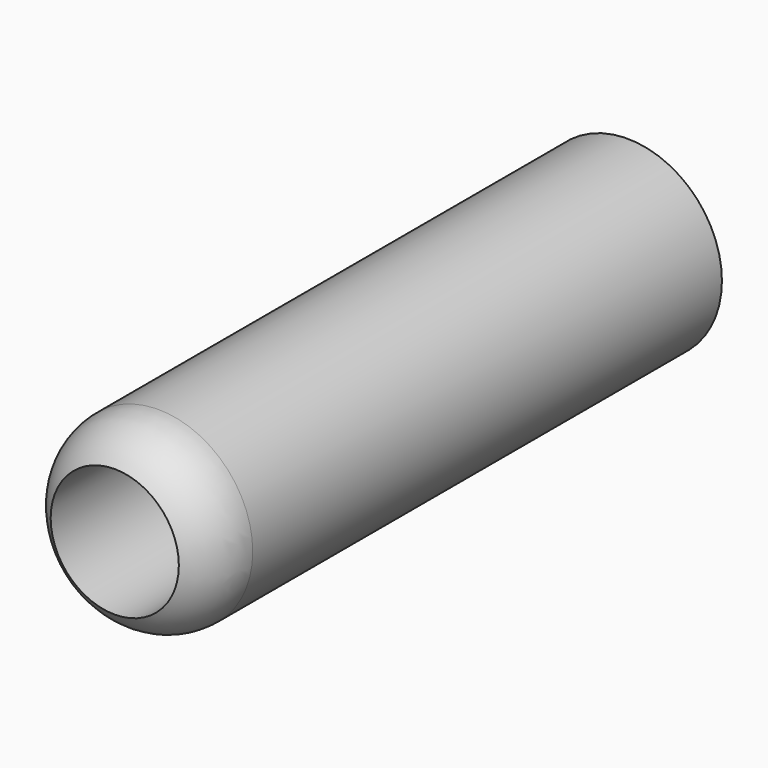
from build123d import *

# Parameters (mm, degrees)
F0_R     = 18.707853832
F1_DEPTH = 127
F3_D     = 25.4


# Not quite as in the source:
# - a fillet or chamfer that OpenCascade refuses, or shapes differently, is made with other operations: its cross-section is extruded or revolved along the edge and cut away or added


with BuildPart() as f1:
    # F0 (on Front) → F1 (new body)
    with BuildSketch(Plane.XZ):
        Circle(F0_R)
    extrude(amount=-F1_DEPTH)

    # F3 (through all)
    with Locations(Plane.XZ):
        with Locations((0, 0)):
            Hole(F3_D / 2)

    # F4: fillet of radius 12.7 on 1 edges, made by hand

    # F4_s1 → F4_t2 (revolve, cut)
    with BuildSketch(Plane.XY):
        with BuildLine():
            ThreePointArc((18.707853832, 10.7937565132), (17.1047060058, 4.6171982618), (12.7, 0))
            Line((12.7, 0), (18.707853832, 0))
            Line((18.707853832, 0), (18.707853832, 10.7937565132))
        make_face()
    revolve(axis=Axis((0, 0, 0), (0, -1, 0)), mode=Mode.SUBTRACT)


solid = f1.part
